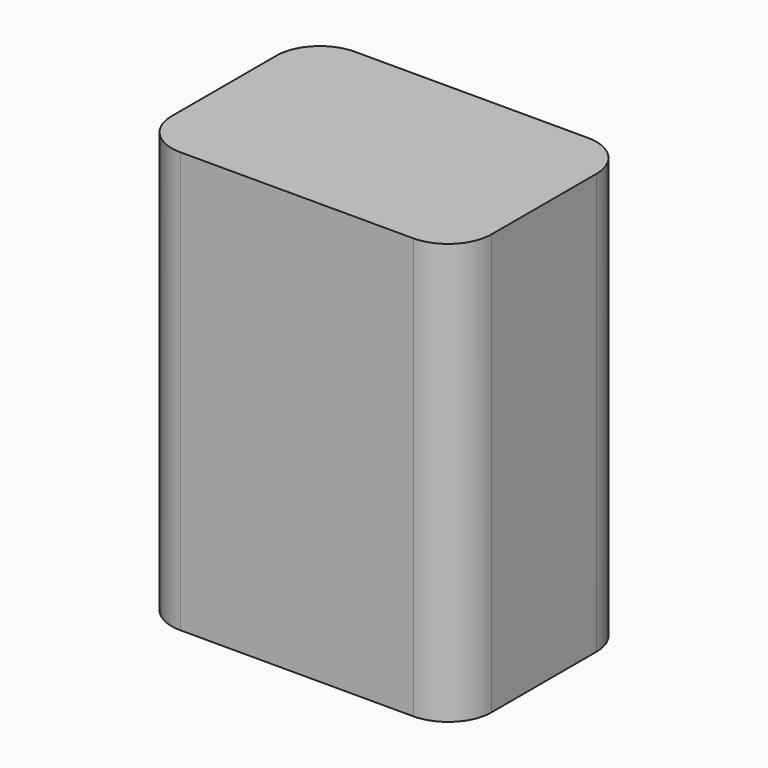
from build123d import *

# Parameters (mm, degrees)
F0_W     = 58.5621017963
F0_H     = 77.0259462297
F1_DEPTH = 39.878
F2_R     = 7.971733183
F3_R     = 6.2062238441
F6_DEPTH = 0.762


# Not quite as in the source:
# - the program builds the solid bodies; features that only make, move or delete a surface that nothing else refers to are left out


with BuildPart() as f1:
    # F0 (on Front) → F1 (new body)
    with BuildSketch(Plane.XZ):
        with Locations((0.5595115945, 2.331295982)):
            Rectangle(F0_W, F0_H)
    extrude(amount=F1_DEPTH)

    # F2
    f2_edges = [f1.edges().sort_by_distance(p)[0] for p in [
        (29.840562, -39.878, 2.331296),
        (-28.721539, -39.878, 2.331296),
        (29.840562, 0, 2.331296),
        (-28.721539, 0, 2.331296),
    ]]
    fillet(f2_edges, radius=F2_R)

    # F3 (on face) → F6 (join)
    with BuildSketch(Plane.XY.offset(40.8442690969)):
        with BuildLine():
            Line((15.5188293097, -6.3193492971), (-17.34697557, -6.3193492971))
            ThreePointArc((-17.34697557, -6.3193492971), (-21.8371036305, -8.1792212365), (-23.69697557, -12.6693492971))
            Line((-23.69697557, -12.6693492971), (-23.69697557, -25.556266817))
            ThreePointArc((-23.69697557, -25.556266817), (-21.8371036305, -30.0463948776), (-17.34697557, -31.906266817))
            Line((-17.34697557, -31.906266817), (15.5188293097, -31.906266817))
            ThreePointArc((15.5188293097, -31.906266817), (20.0089573702, -30.0463948776), (21.8688293097, -25.556266817))
            Line((21.8688293097, -25.556266817), (21.8688293097, -12.6693492971))
            ThreePointArc((21.8688293097, -12.6693492971), (20.0089573702, -8.1792212365), (15.5188293097, -6.3193492971))
        make_face()
        Polygon((-8.0732123646, -19.3963646889), (-10.657480345, -23.8724481314), (-15.826016306, -23.8724481314), (-18.4102842865, -19.3963646889), (-15.826016306, -14.9202812463), (-10.657480345, -14.9202812463), align=None, mode=Mode.SUBTRACT)
        with Locations((8.9521687478, -19.2098617554)):
            Circle(F3_R, mode=Mode.SUBTRACT)
    extrude(amount=-F6_DEPTH)


solid = f1.part
